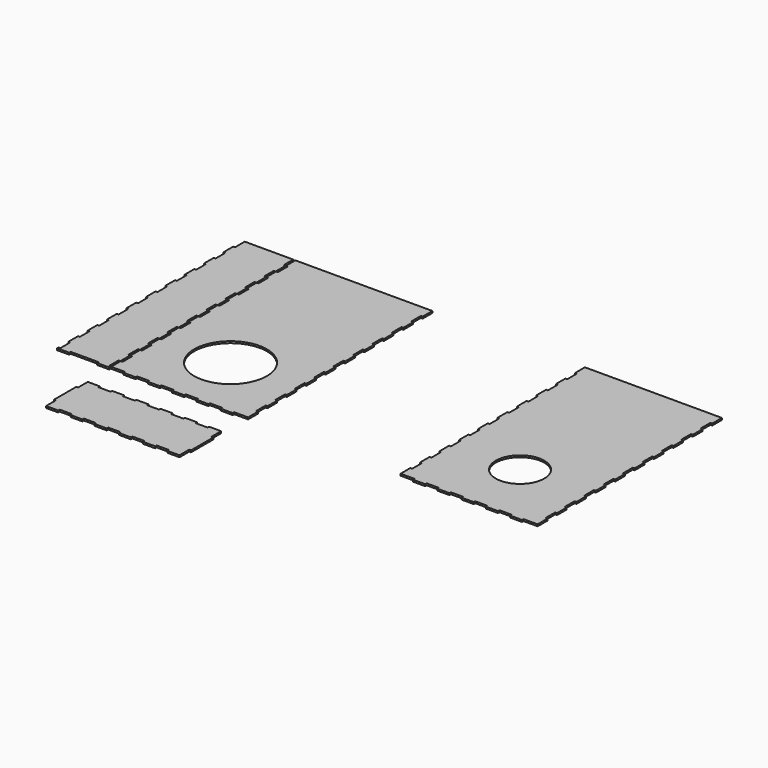
from build123d import *

# Parameters (mm, degrees)
F0_W     = 3
F0_H     = 20
F0_W_2   = 20
F0_H_2   = 3
F1_DEPTH = 3
F0_W_3   = 17
F0_H_3   = 46


# Not quite as in the source:
# - a feature names something its author has since deleted; it is built from what else it names


with BuildPart() as f1:
    # F0 (on Top) → F1 (new body)
    with BuildSketch(Plane.XY):
        with Locations((111.5, -95)):
            Rectangle(F0_W, F0_H)
        with Locations((111.5, -55)):
            Rectangle(F0_W, F0_H)
        with Locations((111.5, -15)):
            Rectangle(F0_W, F0_H)
        with Locations((111.5, 25)):
            Rectangle(F0_W, F0_H)
        with Locations((111.5, 65)):
            Rectangle(F0_W, F0_H)
        with Locations((111.5, 105)):
            Rectangle(F0_W, F0_H)
        with Locations((111.5, 145)):
            Rectangle(F0_W, F0_H)
        with Locations((111.5, 185)):
            Rectangle(F0_W, F0_H)
        with Locations((111.5, 225)):
            Rectangle(F0_W, F0_H)
        with Locations((111.5, 265)):
            Rectangle(F0_W, F0_H)
        with Locations((-111.5, -95)):
            Rectangle(F0_W, F0_H)
        with Locations((-111.5, 265)):
            Rectangle(F0_W, F0_H)
        with Locations((-111.5, -15)):
            Rectangle(F0_W, F0_H)
        with Locations((-111.5, 185)):
            Rectangle(F0_W, F0_H)
        with Locations((-111.5, 145)):
            Rectangle(F0_W, F0_H)
        with Locations((-111.5, 25)):
            Rectangle(F0_W, F0_H)
        with Locations((-111.5, -55)):
            Rectangle(F0_W, F0_H)
        with Locations((-111.5, 105)):
            Rectangle(F0_W, F0_H)
        with Locations((-111.5, 65)):
            Rectangle(F0_W, F0_H)
        with Locations((-111.5, 225)):
            Rectangle(F0_W, F0_H)
        with BuildLine():
            ThreePointArc((0, 60), (42.4264068712, 42.4264068712), (60, 0))
            ThreePointArc((60, 0), (42.4264068712, -42.4264068712), (0, -60))
            Line((0, -60), (0, -105))
            Line((0, -105), (10, -105))
            Line((10, -105), (30, -105))
            Line((30, -105), (50, -105))
            Line((50, -105), (70, -105))
            Line((70, -105), (90, -105))
            Line((90, -105), (110, -105))
            Line((110, -105), (110, -85))
            Line((110, -85), (110, -65))
            Line((110, -65), (110, -45))
            Line((110, -45), (110, -25))
            Line((110, -25), (110, -5))
            Line((110, -5), (110, 15))
            Line((110, 15), (110, 35))
            Line((110, 35), (110, 55))
            Line((110, 55), (110, 75))
            Line((110, 75), (110, 95))
            Line((110, 95), (110, 115))
            Line((110, 115), (110, 135))
            Line((110, 135), (110, 155))
            Line((110, 155), (110, 175))
            Line((110, 175), (110, 195))
            Line((110, 195), (110, 215))
            Line((110, 215), (110, 235))
            Line((110, 235), (110, 255))
            Line((110, 255), (110, 275))
            Line((110, 275), (0, 275))
            Line((0, 275), (0, 60))
        make_face()
        with Locations((40, -106.5)):
            Rectangle(F0_W_2, F0_H_2)
        with Locations((80, -106.5)):
            Rectangle(F0_W_2, F0_H_2)
        with Locations((-80, -106.5)):
            Rectangle(F0_W_2, F0_H_2)
        with Locations((-40, -106.5)):
            Rectangle(F0_W_2, F0_H_2)
        Polygon((10, -105), (0, -105), (-10, -105), (-10, -108), (10, -108), align=None)
        with BuildLine():
            ThreePointArc((0, -60), (-60, 0), (0, 60))
            Line((0, 60), (0, 275))
            Line((0, 275), (-110, 275))
            Line((-110, 275), (-110, 255))
            Line((-110, 255), (-110, 235))
            Line((-110, 235), (-110, 215))
            Line((-110, 215), (-110, 195))
            Line((-110, 195), (-110, 175))
            Line((-110, 175), (-110, 155))
            Line((-110, 155), (-110, 135))
            Line((-110, 135), (-110, 115))
            Line((-110, 115), (-110, 95))
            Line((-110, 95), (-110, 75))
            Line((-110, 75), (-110, 55))
            Line((-110, 55), (-110, 35))
            Line((-110, 35), (-110, 15))
            Line((-110, 15), (-110, -5))
            Line((-110, -5), (-110, -25))
            Line((-110, -25), (-110, -45))
            Line((-110, -45), (-110, -65))
            Line((-110, -65), (-110, -85))
            Line((-110, -85), (-110, -105))
            Line((-110, -105), (-90, -105))
            Line((-90, -105), (-70, -105))
            Line((-70, -105), (-50, -105))
            Line((-50, -105), (-30, -105))
            Line((-30, -105), (-10, -105))
            Line((-10, -105), (0, -105))
            Line((0, -105), (0, -60))
        make_face()
    extrude(amount=F1_DEPTH)


with BuildPart() as f1b:
    # F0 (on Top) → F1, piece 2 (new body)
    with BuildSketch(Plane.XY):
        Polygon((-179.5, -105), (-156.5, -105), (-156.5, 275), (-196.5, 275), (-196.5, 255), (-196.5, 235), (-196.5, 215), (-196.5, 195), (-196.5, 175), (-196.5, 155), (-196.5, 135), (-196.5, 115), (-196.5, 95), (-196.5, 75), (-196.5, 55), (-196.5, 35), (-196.5, 15), (-196.5, -5), (-196.5, -25), (-196.5, -45), (-196.5, -65), (-196.5, -85), (-196.5, -105), align=None)
        with Locations((-115, 85)):
            Rectangle(F0_W, F0_H)
        with Locations((-198, 85)):
            Rectangle(F0_W, F0_H)
        with Locations((-115, 165)):
            Rectangle(F0_W, F0_H)
        with Locations((-115, 45)):
            Rectangle(F0_W, F0_H)
        with Locations((-115, 125)):
            Rectangle(F0_W, F0_H)
        with Locations((-115, 205)):
            Rectangle(F0_W, F0_H)
        with Locations((-115, -75)):
            Rectangle(F0_W, F0_H)
        with Locations((-115, 5)):
            Rectangle(F0_W, F0_H)
        with Locations((-115, 245)):
            Rectangle(F0_W, F0_H)
        with Locations((-115, -35)):
            Rectangle(F0_W, F0_H)
        with Locations((-198, 5)):
            Rectangle(F0_W, F0_H)
        with Locations((-198, 245)):
            Rectangle(F0_W, F0_H)
        with Locations((-198, 205)):
            Rectangle(F0_W, F0_H)
        with Locations((-198, -35)):
            Rectangle(F0_W, F0_H)
        with Locations((-198, 45)):
            Rectangle(F0_W, F0_H)
        with Locations((-198, -75)):
            Rectangle(F0_W, F0_H)
        with Locations((-198, 165)):
            Rectangle(F0_W, F0_H)
        with Locations((-198, 125)):
            Rectangle(F0_W, F0_H)
        Polygon((-156.5, 275), (-156.5, -105), (-133.5, -105), (-116.5, -105), (-116.5, -85), (-116.5, -65), (-116.5, -45), (-116.5, -25), (-116.5, -5), (-116.5, 15), (-116.5, 35), (-116.5, 55), (-116.5, 75), (-116.5, 95), (-116.5, 115), (-116.5, 135), (-116.5, 155), (-116.5, 175), (-116.5, 195), (-116.5, 215), (-116.5, 235), (-116.5, 255), (-116.5, 275), align=None)
        with Locations((-188, -106.5)):
            Rectangle(F0_W_3, F0_H_2)
        with Locations((-198, -106.5)):
            Rectangle(F0_W, F0_H_2)
        with Locations((-125, -106.5)):
            Rectangle(F0_W_3, F0_H_2)
        with Locations((-115, -106.5)):
            Rectangle(F0_W, F0_H_2)
    extrude(amount=F1_DEPTH)


with BuildPart() as f1c:
    # F0 (on Top) → F1, piece 3 (new body)
    with BuildSketch(Plane.XY):
        Polygon((-90, -159.7509366274), (-110, -159.7509366274), (-110, -176.7509366274), (-110, -222.7509366274), (-110, -239.7509366274), (-90, -239.7509366274), (-70, -239.7509366274), (-50, -239.7509366274), (-30, -239.7509366274), (-10, -239.7509366274), (10, -239.7509366274), (30, -239.7509366274), (50, -239.7509366274), (70, -239.7509366274), (90, -239.7509366274), (110, -239.7509366274), (110, -222.7509366274), (110, -176.7509366274), (110, -159.7509366274), (90, -159.7509366274), (70, -159.7509366274), (50, -159.7509366274), (30, -159.7509366274), (10, -159.7509366274), (-10, -159.7509366274), (-30, -159.7509366274), (-50, -159.7509366274), (-70, -159.7509366274), align=None)
        with Locations((-20, -241.2509366274)):
            Rectangle(F0_W_2, F0_H_2)
        with Locations((20, -241.2509366274)):
            Rectangle(F0_W_2, F0_H_2)
        with Locations((60, -241.2509366274)):
            Rectangle(F0_W_2, F0_H_2)
        with Locations((-60, -241.2509366274)):
            Rectangle(F0_W_2, F0_H_2)
        with Locations((-100, -241.2509366274)):
            Rectangle(F0_W_2, F0_H_2)
        with Locations((100, -241.2509366274)):
            Rectangle(F0_W_2, F0_H_2)
        with Locations((111.5, -199.7509366274)):
            Rectangle(F0_W, F0_H_3)
        with Locations((-20, -158.2509366274)):
            Rectangle(F0_W_2, F0_H_2)
        with Locations((20, -158.2509366274)):
            Rectangle(F0_W_2, F0_H_2)
        with Locations((60, -158.2509366274)):
            Rectangle(F0_W_2, F0_H_2)
        with Locations((100, -158.2509366274)):
            Rectangle(F0_W_2, F0_H_2)
        with Locations((-100, -158.2509366274)):
            Rectangle(F0_W_2, F0_H_2)
        with Locations((-111.5, -199.7509366274)):
            Rectangle(F0_W, F0_H_3)
        with Locations((-60, -158.2509366274)):
            Rectangle(F0_W_2, F0_H_2)
    extrude(amount=F1_DEPTH)


with BuildPart() as f1d:
    # F0 (on Top) → F1, piece 4 (new body)
    with BuildSketch(Plane.XY):
        with BuildLine():
            ThreePointArc((477.5, -40), (437.5, 0), (477.5, 40))
            Line((477.5, 40), (477.5, 275))
            Line((477.5, 275), (367.5, 275))
            Line((367.5, 275), (367.5, 255))
            Line((367.5, 255), (367.5, 235))
            Line((367.5, 235), (367.5, 215))
            Line((367.5, 215), (367.5, 195))
            Line((367.5, 195), (367.5, 175))
            Line((367.5, 175), (367.5, 155))
            Line((367.5, 155), (367.5, 135))
            Line((367.5, 135), (367.5, 115))
            Line((367.5, 115), (367.5, 95))
            Line((367.5, 95), (367.5, 75))
            Line((367.5, 75), (367.5, 55))
            Line((367.5, 55), (367.5, 35))
            Line((367.5, 35), (367.5, 15))
            Line((367.5, 15), (367.5, -5))
            Line((367.5, -5), (367.5, -25))
            Line((367.5, -25), (367.5, -45))
            Line((367.5, -45), (367.5, -65))
            Line((367.5, -65), (367.5, -85))
            Line((367.5, -85), (367.5, -105))
            Line((367.5, -105), (387.5, -105))
            Line((387.5, -105), (407.5, -105))
            Line((407.5, -105), (427.5, -105))
            Line((427.5, -105), (447.5, -105))
            Line((447.5, -105), (467.5, -105))
            Line((467.5, -105), (477.5, -105))
            Line((477.5, -105), (477.5, -40))
        make_face()
        with BuildLine():
            ThreePointArc((477.5, 40), (505.7842712475, 28.2842712475), (517.5, 0))
            ThreePointArc((517.5, 0), (505.7842712475, -28.2842712475), (477.5, -40))
            Line((477.5, -40), (477.5, -105))
            Line((477.5, -105), (487.5, -105))
            Line((487.5, -105), (507.5, -105))
            Line((507.5, -105), (527.5, -105))
            Line((527.5, -105), (547.5, -105))
            Line((547.5, -105), (567.5, -105))
            Line((567.5, -105), (587.5, -105))
            Line((587.5, -105), (587.5, -85))
            Line((587.5, -85), (587.5, -65))
            Line((587.5, -65), (587.5, -45))
            Line((587.5, -45), (587.5, -25))
            Line((587.5, -25), (587.5, -5))
            Line((587.5, -5), (587.5, 15))
            Line((587.5, 15), (587.5, 35))
            Line((587.5, 35), (587.5, 55))
            Line((587.5, 55), (587.5, 75))
            Line((587.5, 75), (587.5, 95))
            Line((587.5, 95), (587.5, 115))
            Line((587.5, 115), (587.5, 135))
            Line((587.5, 135), (587.5, 155))
            Line((587.5, 155), (587.5, 175))
            Line((587.5, 175), (587.5, 195))
            Line((587.5, 195), (587.5, 215))
            Line((587.5, 215), (587.5, 235))
            Line((587.5, 235), (587.5, 255))
            Line((587.5, 255), (587.5, 275))
            Line((587.5, 275), (477.5, 275))
            Line((477.5, 275), (477.5, 40))
        make_face()
        with Locations((366, 105)):
            Rectangle(F0_W, F0_H)
        with Locations((366, 185)):
            Rectangle(F0_W, F0_H)
        with Locations((366, 225)):
            Rectangle(F0_W, F0_H)
        with Locations((589, 65)):
            Rectangle(F0_W, F0_H)
        with Locations((397.5, -106.5)):
            Rectangle(F0_W_2, F0_H_2)
        with Locations((437.5, -106.5)):
            Rectangle(F0_W_2, F0_H_2)
        with Locations((517.5, -106.5)):
            Rectangle(F0_W_2, F0_H_2)
        with Locations((589, -95)):
            Rectangle(F0_W, F0_H)
        with Locations((589, 265)):
            Rectangle(F0_W, F0_H)
        with Locations((589, 185)):
            Rectangle(F0_W, F0_H)
        with Locations((589, 145)):
            Rectangle(F0_W, F0_H)
        with Locations((557.5, -106.5)):
            Rectangle(F0_W_2, F0_H_2)
        with Locations((589, -55)):
            Rectangle(F0_W, F0_H)
        with Locations((366, -15)):
            Rectangle(F0_W, F0_H)
        with Locations((366, 65)):
            Rectangle(F0_W, F0_H)
        with Locations((366, -55)):
            Rectangle(F0_W, F0_H)
        with Locations((589, 105)):
            Rectangle(F0_W, F0_H)
        with Locations((366, 265)):
            Rectangle(F0_W, F0_H)
        with Locations((589, -15)):
            Rectangle(F0_W, F0_H)
        with Locations((366, 25)):
            Rectangle(F0_W, F0_H)
        with Locations((589, 25)):
            Rectangle(F0_W, F0_H)
        with Locations((366, 145)):
            Rectangle(F0_W, F0_H)
        Polygon((487.5, -105), (477.5, -105), (467.5, -105), (467.5, -108), (487.5, -108), align=None)
        with Locations((589, 225)):
            Rectangle(F0_W, F0_H)
        with Locations((366, -95)):
            Rectangle(F0_W, F0_H)
    extrude(amount=F1_DEPTH)


solid = Compound([f1.part, f1b.part, f1c.part, f1d.part])
